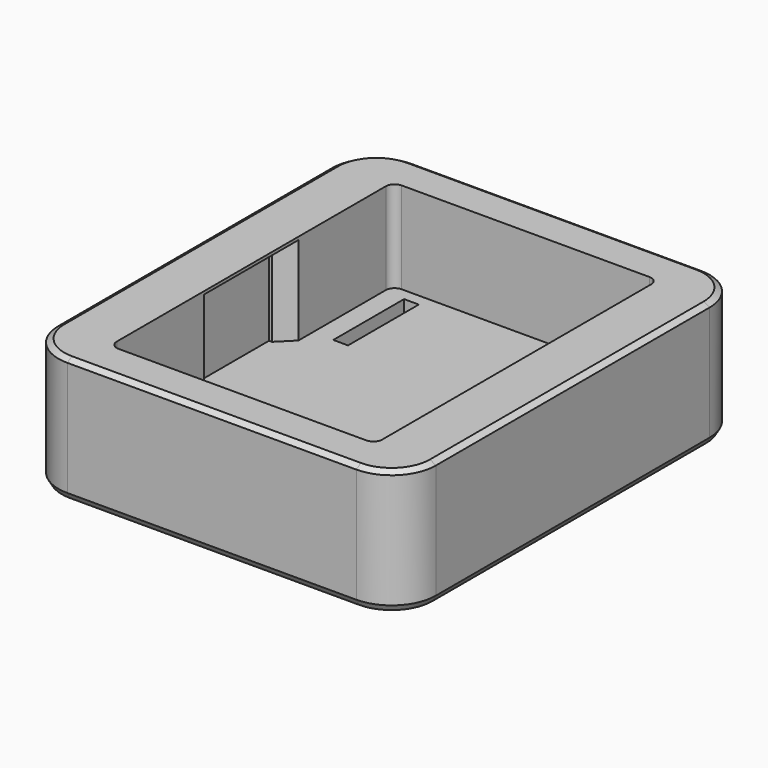
from build123d import *

# Parameters (mm, degrees)
F0_W          = 64
F0_H          = 73
F1_DEPTH      = 5.5
F2_DEPTH      = 15.5
F3_W          = 15
F3_H          = 0.5
F4_DEPTH      = 3
F6_W          = 2.5
F6_H          = 15
F7_DEPTH      = 5.501
F8_SIZE       = 2.5
F9_R          = 1.5
F10_R         = 7.5
F11_T1_DEPTH  = 58
F11_T3_DEPTH  = 49
F11_T5_DEPTH  = 2.5
F11_T7_DEPTH  = 15
F11_T10_ANGLE = 90
F11_T12_ANGLE = 90
F11_T14_ANGLE = 90
F11_T16_ANGLE = 90
F11_T21_DEPTH = 5.0870857546
F11_T25_DEPTH = 17.5870857546
F11_T32_DEPTH = 5.0870857546
F11_T36_DEPTH = 17.5870857546
F11_T43_DEPTH = 17.5870857546
F11_T47_DEPTH = 5.0870857546
F11_T54_DEPTH = 5.0870857546
F11_T58_DEPTH = 17.5870857546
F12_SIZE2     = 0.5773502692
F12_SIZE      = 1


# Not quite as in the source:
# - a fillet or chamfer that OpenCascade refuses, or shapes differently, is made with other operations: its cross-section is extruded or revolved along the edge and cut away or added


with BuildPart() as f1:
    # F0 (on Top) → F1 (new body)
    with BuildSketch(Plane.XY):
        Rectangle(F0_W, F0_H)
        Polygon((-22.5, 7.5), (-22.5, 30), (22.5, 30), (22.5, 7.5), (25.5, 7.5), (25.5, -7.5), (22.5, -7.5), (22.5, -30), (-22.5, -30), (-22.5, -7.5), (-25.5, -7.5), (-25.5, 7.5), align=None, mode=Mode.SUBTRACT)
        Polygon((22.5, 30), (-22.5, 30), (-22.5, 7.5), (-25.5, 7.5), (-25.5, -7.5), (-22.5, -7.5), (-22.5, -30), (22.5, -30), (22.5, -7.5), (25.5, -7.5), (25.5, 7.5), (22.5, 7.5), align=None)
    extrude(amount=-F1_DEPTH)

    # F0 (on Top) → F2 (join)
    with BuildSketch(Plane.XY):
        Rectangle(F0_W, F0_H)
        Polygon((-22.5, 7.5), (-22.5, 30), (22.5, 30), (22.5, 7.5), (25.5, 7.5), (25.5, -7.5), (22.5, -7.5), (22.5, -30), (-22.5, -30), (-22.5, -7.5), (-25.5, -7.5), (-25.5, 7.5), align=None, mode=Mode.SUBTRACT)
    extrude(amount=F2_DEPTH)

    # F3 (on face) → F4 (join, through all)
    with BuildSketch(Plane.YZ.offset(-25.5)):
        with Locations((0, 15.25)):
            Rectangle(F3_W, F3_H)
    extrude(amount=F4_DEPTH)

    # F5: F1 across plane


with BuildPart() as f1_1:
    add(f1.part)
    add(f1.part.mirror(Plane.YZ))

    # F6 (on face) → F7 (cut, through all)
    with BuildSketch(Plane.XY):
        with Locations((-17.75, 20.5)):
            Rectangle(F6_W, F6_H)
    extrude(amount=-F7_DEPTH, mode=Mode.SUBTRACT)

    # F8
    f8_edges = [f1_1.edges().sort_by_distance(p)[0] for p in [
        (-22.5, -7.5, 7.5),
        (-22.5, 7.5, 7.5),
        (22.5, 7.5, 7.5),
        (22.5, -7.5, 7.5),
    ]]
    chamfer(f8_edges, length=F8_SIZE)

    # F9
    f9_edges = [f1_1.edges().sort_by_distance(p)[0] for p in [
        (-22.5, 30, 7.75),
        (-22.5, -30, 7.75),
        (22.5, 30, 7.75),
        (22.5, -30, 7.75),
    ]]
    fillet(f9_edges, radius=F9_R)

    # F10
    f10_edges = [f1_1.edges().sort_by_distance(p)[0] for p in [
        (-32, -36.5, 5),
        (32, -36.5, 5),
        (-32, 36.5, 5),
        (32, 36.5, 5),
    ]]
    fillet(f10_edges, radius=F10_R)

    # F11: chamfer of 1 x 0.5773502692 on 12 edges, made by hand

    # F11_s2 → F11_t1 (cut)
    with BuildSketch(Plane.XZ.offset(-29)):
        Polygon((32, -4.5), (31.4226497308, -5.5), (32, -5.5), align=None)
        Polygon((-32, -4.5), (-31.4226497308, -5.5), (-32, -5.5), align=None)
    extrude(amount=F11_T1_DEPTH, mode=Mode.SUBTRACT)

    # F11_s4 → F11_t3 (cut)
    with BuildSketch(Plane.YZ.offset(-24.5)):
        Polygon((-36.5, -4.5), (-35.9226497308, -5.5), (-36.5, -5.5), align=None)
        Polygon((36.5, -4.5), (35.9226497308, -5.5), (36.5, -5.5), align=None)
    extrude(amount=F11_T3_DEPTH, mode=Mode.SUBTRACT)

    # F11_s6 → F11_t5 (cut)
    with BuildSketch(Plane.YZ.offset(-19)):
        Polygon((28.5773502692, -5.5), (28, -4.5), (28, -5.5), align=None)
        Polygon((12.4226497308, -5.5), (13, -4.5), (13, -5.5), align=None)
    extrude(amount=F11_T5_DEPTH, mode=Mode.SUBTRACT)

    # F11_s8 → F11_t7 (cut)
    with BuildSketch(Plane.XZ.offset(-28)):
        Polygon((-19.5773502692, -5.5), (-19, -4.5), (-19, -5.5), align=None)
        Polygon((-15.9226497308, -5.5), (-16.5, -4.5), (-16.5, -5.5), align=None)
    extrude(amount=F11_T7_DEPTH, mode=Mode.SUBTRACT)

    # F11_s9 → F11_t10 (revolve, cut)
    with BuildSketch(Plane.XZ.offset(29)):
        Polygon((32, -4.5), (31.4226497308, -5.5), (32, -5.5), align=None)
    revolve(axis=Axis((24.5, -29, -5.5), (0, 0, -1)), revolution_arc=F11_T10_ANGLE, mode=Mode.SUBTRACT)

    # F11_s11 → F11_t12 (revolve, cut)
    with BuildSketch(Plane.XZ.offset(-29)):
        Polygon((32, -4.5), (31.4226497308, -5.5), (32, -5.5), align=None)
    revolve(axis=Axis((24.5, 29, -5.5), (0, 0, 1)), revolution_arc=F11_T12_ANGLE, mode=Mode.SUBTRACT)

    # F11_s13 → F11_t14 (revolve, cut)
    with BuildSketch(Plane.XZ.offset(29)):
        Polygon((-32, -4.5), (-31.4226497308, -5.5), (-32, -5.5), align=None)
    revolve(axis=Axis((-24.5, -29, -5.5), (0, 0, 1)), revolution_arc=F11_T14_ANGLE, mode=Mode.SUBTRACT)

    # F11_s15 → F11_t16 (revolve, cut)
    with BuildSketch(Plane.YZ.offset(-24.5)):
        Polygon((36.5, -4.5), (35.9226497308, -5.5), (36.5, -5.5), align=None)
    revolve(axis=Axis((-24.5, 29, -5.5), (0, 0, 1)), revolution_arc=F11_T16_ANGLE, mode=Mode.SUBTRACT)


with BuildPart() as f11_tool19:
    # F11_s20 → F11_t21 (new body)
    with BuildSketch(Plane.YZ.offset(-13.9129142454)):
        Polygon((28.5773502692, -5.5), (28, -4.5), (28, -5.5), align=None)
    extrude(amount=-F11_T21_DEPTH)

    split(bisect_by=Plane.YZ.offset(-16.5), keep=Keep.TOP)


with BuildPart() as f11_tool23:
    # F11_s24 → F11_t25 (new body)
    with BuildSketch(Plane.XZ.offset(-13)):
        Polygon((-15.9226497308, -5.5), (-16.5, -4.5), (-16.5, -5.5), align=None)
    extrude(amount=-F11_T25_DEPTH)

    split(bisect_by=Plane.XZ.offset(-28), keep=Keep.BOTTOM)


with BuildPart() as f11_tool19_1:
    add(f11_tool19.part)

    # F11_t27: intersect F11_tool23
    add(f11_tool23.part, mode=Mode.INTERSECT)


with BuildPart() as f1_2:
    add(f1_1.part)

    # F11_t17: cut F11_tool19
    add(f11_tool19_1.part, mode=Mode.SUBTRACT)


with BuildPart() as f11_tool30:
    # F11_s31 → F11_t32 (new body)
    with BuildSketch(Plane.YZ.offset(-16.5)):
        Polygon((28.5773502692, -5.5), (28, -4.5), (28, -5.5), align=None)
    extrude(amount=-F11_T32_DEPTH)

    split(bisect_by=Plane.YZ.offset(-19), keep=Keep.BOTTOM)


with BuildPart() as f11_tool34:
    # F11_s35 → F11_t36 (new body)
    with BuildSketch(Plane.XZ.offset(-30.5870857546)):
        Polygon((-19.5773502692, -5.5), (-19, -4.5), (-19, -5.5), align=None)
    extrude(amount=F11_T36_DEPTH)

    split(bisect_by=Plane.XZ.offset(-28), keep=Keep.BOTTOM)


with BuildPart() as f11_tool30_1:
    add(f11_tool30.part)

    # F11_t38: intersect F11_tool34
    add(f11_tool34.part, mode=Mode.INTERSECT)


with BuildPart() as f1_3:
    add(f1_2.part)

    # F11_t28: cut F11_tool30
    add(f11_tool30_1.part, mode=Mode.SUBTRACT)


with BuildPart() as f11_tool41:
    # F11_s42 → F11_t43 (new body)
    with BuildSketch(Plane.XZ.offset(-28)):
        Polygon((-19.5773502692, -5.5), (-19, -4.5), (-19, -5.5), align=None)
    extrude(amount=F11_T43_DEPTH)

    split(bisect_by=Plane.XZ.offset(-13), keep=Keep.TOP)


with BuildPart() as f11_tool45:
    # F11_s46 → F11_t47 (new body)
    with BuildSketch(Plane.YZ.offset(-21.5870857546)):
        Polygon((12.4226497308, -5.5), (13, -4.5), (13, -5.5), align=None)
    extrude(amount=F11_T47_DEPTH)

    split(bisect_by=Plane.YZ.offset(-19), keep=Keep.BOTTOM)


with BuildPart() as f11_tool41_1:
    add(f11_tool41.part)

    # F11_t49: intersect F11_tool45
    add(f11_tool45.part, mode=Mode.INTERSECT)


with BuildPart() as f1_4:
    add(f1_3.part)

    # F11_t39: cut F11_tool41
    add(f11_tool41_1.part, mode=Mode.SUBTRACT)


with BuildPart() as f11_tool52:
    # F11_s53 → F11_t54 (new body)
    with BuildSketch(Plane.YZ.offset(-19)):
        Polygon((12.4226497308, -5.5), (13, -4.5), (13, -5.5), align=None)
    extrude(amount=F11_T54_DEPTH)

    split(bisect_by=Plane.YZ.offset(-16.5), keep=Keep.TOP)


with BuildPart() as f11_tool56:
    # F11_s57 → F11_t58 (new body)
    with BuildSketch(Plane.XZ.offset(-10.4129142454)):
        Polygon((-15.9226497308, -5.5), (-16.5, -4.5), (-16.5, -5.5), align=None)
    extrude(amount=-F11_T58_DEPTH)

    split(bisect_by=Plane.XZ.offset(-13), keep=Keep.TOP)


with BuildPart() as f11_tool52_1:
    add(f11_tool52.part)

    # F11_t60: intersect F11_tool56
    add(f11_tool56.part, mode=Mode.INTERSECT)


with BuildPart() as f1_5:
    add(f1_4.part)

    # F11_t50: cut F11_tool52
    add(f11_tool52_1.part, mode=Mode.SUBTRACT)

    # F12
    f12_edges = [f1_5.edges().sort_by_distance(p)[0] for p in [
        (-29.803301, -34.303301, 15.5),
        (-32, 0, 15.5),
        (0, -36.5, 15.5),
        (29.803301, -34.303301, 15.5),
        (32, 0, 15.5),
        (29.803301, 34.303301, 15.5),
        (0, 36.5, 15.5),
        (-29.803301, 34.303301, 15.5),
    ]]
    chamfer(f12_edges, length=F12_SIZE, length2=F12_SIZE2)


solid = f1_5.part
